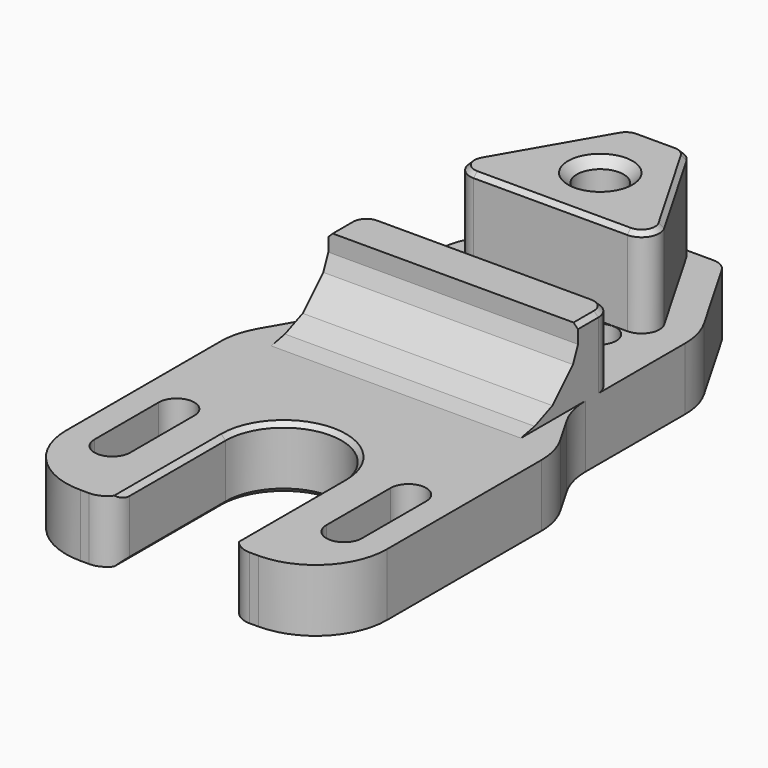
from build123d import *

# Parameters (mm, degrees)
F1_DEPTH      = 10
F3_DEPTH      = 7
F4_R          = 2.615
F4_W          = 5
F4_H          = 10
F5_DEPTH      = 10.001
F5_DEPTH_BACK = 25
F6_W          = 28
F6_H          = 7
F7_DEPTH      = 50
F8_W          = 28
F8_H          = 5
F9_DEPTH      = 8
F10_SIZE      = 5
F11_SIZE      = 2
F12_SIZE      = 1
F13_SIZE      = 1
F14_R         = 8
F15_SIZE      = 1
F17_DEPTH     = 10.001
F18_R         = 2
F20_DEPTH     = 7.001
F22_DEPTH     = 7
F23_R         = 8
F25_DEPTH     = 7.001
F26_SIZE      = 0.5
F27_R         = 1.99
F28_DEPTH     = 17.001
F29_R         = 2.5


# Not quite as in the source:
# - a feature names something its author has since deleted; it is built from what else it names


with BuildPart() as f1:
    # F0 (on Top) → F1 (new body)
    with BuildSketch(Plane.XY):
        Polygon((0, 14.2484272933), (-12.3395, -7.1242136467), (12.3395, -7.1242136467), align=None)
    extrude(amount=F1_DEPTH)

    # F2 (on face) → F3 (join)
    with BuildSketch(Plane(origin=(0, 0, 0), x_dir=(1, 0, 0), z_dir=(0, 0, -1))):
        Polygon((-18, 10.3923048454), (0, -20.7846096908), (18, 10.3923048454), align=None)
    extrude(amount=F3_DEPTH)

    # F4 (on Top) → F5 (cut, two sides)
    with BuildSketch(Plane.XY) as f5_sk:
        Polygon((-11.5514649078, 20.9689907423), (-11.4649338648, 8.2484272933), (13.3285973679, 8.2484272933), (13.3285973679, 20.9689907423), align=None)
        Circle(F4_R)
        with Locations((-16.5, -8)):
            Rectangle(F4_W, F4_H)
        with Locations((16.5, -8)):
            Rectangle(F4_W, F4_H)
    extrude(amount=F5_DEPTH, mode=Mode.SUBTRACT)
    extrude(f5_sk.sketch, amount=-F5_DEPTH_BACK, mode=Mode.SUBTRACT)

    # F6 (on face) → F7 (join)
    with BuildSketch(Plane.XZ.offset(10.3923048454)):
        with Locations((0, -3.5)):
            Rectangle(F6_W, F6_H)
    extrude(amount=F7_DEPTH)

    # F8 (on face) → F9 (join)
    with BuildSketch(Plane.XY):
        with Locations((0, -18.1242136467)):
            Rectangle(F8_W, F8_H)
    extrude(amount=F9_DEPTH)

    # F10
    f10_edges = [f1.edges().sort_by_distance(p)[0] for p in [
        (0, -20.624214, 0),
    ]]
    chamfer(f10_edges, length=F10_SIZE)

    # F11
    f11_edges = [f1.edges().sort_by_distance(p)[0] for p in [
        (0, -25.624214, 0),
    ]]
    chamfer(f11_edges, length=F11_SIZE)

    # F12
    f12_edges = [f1.edges().sort_by_distance(p)[0] for p in [
        (0, -27.624214, 0),
    ]]
    chamfer(f12_edges, length=F12_SIZE)

    # F13
    f13_edges = [f1.edges().sort_by_distance(p)[0] for p in [
        (0, -20.624214, 5),
    ]]
    chamfer(f13_edges, length=F13_SIZE)

    # F14
    f14_edges = [f1.edges().sort_by_distance(p)[0] for p in [
        (-14, -3.464102, -3.5),
        (14, -3.464102, -3.5),
    ]]
    fillet(f14_edges, radius=F14_R)

    # F15
    f15_edges = [f1.edges().sort_by_distance(p)[0] for p in [
        (-2.615, 0, 10),
        (-2.615, 0, -7),
    ]]
    chamfer(f15_edges, length=F15_SIZE)

    # F16 (on face) → F17 (cut, through all)
    with BuildSketch(Plane.XY):
        Polygon((12.0796923789, -6.9742136467), (-12.0796923789, -6.9742136467), (-3.2908965344, 8.2484272933), (-14, 8.2484272933), (-14, -15.7742136467), (14, -15.7742136467), (14, 8.2484272933), (7.2377682818, 8.2484272933), (3.2908965344, 8.2484272933), align=None)
    extrude(amount=F17_DEPTH, mode=Mode.SUBTRACT)

    # F18
    f18_edges = [f1.edges().sort_by_distance(p)[0] for p in [
        (-12.079692, -6.974214, 5),
        (12.079692, -6.974214, 5),
        (3.290897, 8.248427, 5),
        (-3.290897, 8.248427, 5),
        (-7.237768, 8.248427, -3.5),
        (7.237768, 8.248427, -3.5),
        (-14, -15.774214, 4),
        (14, -15.774214, 4),
    ]]
    fillet(f18_edges, radius=F18_R)

    # F19 (on face) → F20 (cut, through all)
    with BuildSketch(Plane.XY):
        with BuildLine():
            Line((6.5, -50.8923048454), (6.5, -44.3923048454))
            ThreePointArc((6.5, -44.3923048454), (0, -37.8923048454), (-6.5, -44.3923048454))
            Line((-6.5, -44.3923048454), (-6.5, -50.8923048454))
            Line((-6.5, -50.8923048454), (-6.5, -60.3923048454))
            Line((-6.5, -60.3923048454), (6.5, -60.3923048454))
            Line((6.5, -60.3923048454), (6.5, -50.8923048454))
        make_face()
    extrude(amount=-F20_DEPTH, mode=Mode.SUBTRACT)

    # F21 (on face) → F22 (join, through all)
    with BuildSketch(Plane.XY):
        Polygon((-14, -60.3923048454), (-14, -28.6242136467), (-14, -21.6960104164), (-18, -28.6242136467), (-18, -60.3923048454), align=None)
        Polygon((14, -28.6242136467), (14, -60.3923048454), (18, -60.3923048454), (18, -28.6242136467), (14, -21.6960104164), align=None)
    extrude(amount=-F22_DEPTH)

    # F23
    f23_edges = [f1.edges().sort_by_distance(p)[0] for p in [
        (18, -28.624214, -3.5),
        (14, -21.69601, -3.5),
        (-14, -21.69601, -3.5),
        (-18, -28.624214, -3.5),
        (-18, -60.392305, -3.5),
        (18, -60.392305, -3.5),
    ]]
    fillet(f23_edges, radius=F23_R)

    # F24 (on face) → F25 (cut, through all)
    with BuildSketch(Plane.XY):
        with BuildLine():
            Line((-11, -52.1423048454), (-11, -43.1423048454))
            ThreePointArc((-11, -43.1423048454), (-13, -41.1423048454), (-15, -43.1423048454))
            Line((-15, -43.1423048454), (-15, -52.1423048454))
            ThreePointArc((-15, -52.1423048454), (-13, -54.1423048454), (-11, -52.1423048454))
        make_face()
        with BuildLine():
            Line((15, -52.1423048454), (15, -43.1423048454))
            ThreePointArc((15, -43.1423048454), (13, -41.1423048454), (11, -43.1423048454))
            Line((11, -43.1423048454), (11, -52.1423048454))
            ThreePointArc((11, -52.1423048454), (13, -54.1423048454), (15, -52.1423048454))
        make_face()
    extrude(amount=-F25_DEPTH, mode=Mode.SUBTRACT)

    # F26
    f26_edges = [f1.edges().sort_by_distance(p)[0] for p in [
        (6.5, -52.392305, -7),
        (6.5, -52.392305, 0),
        (0, -6.974214, 10),
        (0, -15.774214, 8),
        (0, -37.892305, -7),
        (-6.5, -52.392305, -7),
        (-11, -47.642305, -7),
        (-13, -54.142305, -7),
        (-15, -47.642305, -7),
        (-13, -41.142305, -7),
        (15, -47.642305, -7),
        (13, -54.142305, -7),
        (11, -47.642305, -7),
        (13, -41.142305, -7),
        (-6.5, -52.392305, 0),
        (0, -37.892305, 0),
        (14, -19.199214, 8),
        (13.414214, -16.36, 8),
        (-14, -19.199214, 8),
        (-13.414214, -16.36, 8),
        (3.136196, 7.980478, 10),
        (7.107944, 1.637107, 10),
        (10.347642, -5.974214, 10),
        (0, 8.248427, 10),
        (-10.347642, -5.974214, 10),
        (-3.136196, 7.980478, 10),
        (-7.107944, 1.637107, 10),
    ]]
    chamfer(f26_edges, length=F26_SIZE)

    # F27 (on face) → F28 (cut, through all)
    with BuildSketch(Plane(origin=(0, 0, -7), x_dir=(1, 0, 0), z_dir=(0, 0, -1))):
        with Locations((-7, 9.0015727067)):
            Circle(F27_R)
        with Locations((7, 9.0015727067)):
            Circle(F27_R)
    extrude(amount=-F28_DEPTH, mode=Mode.SUBTRACT)

    # F29
    f29_edges = [f1.edges().sort_by_distance(p)[0] for p in [
        (-6.5, -60.392305, -3.5),
        (6.5, -60.392305, -3.5),
    ]]
    fillet(f29_edges, radius=F29_R)


solid = f1.part
